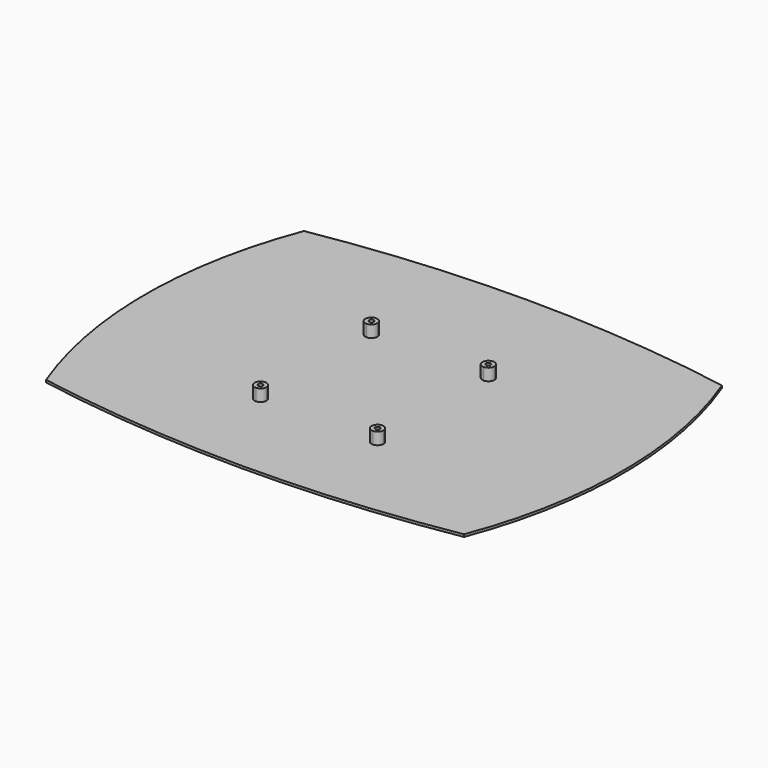
from build123d import *

# Parameters (mm, degrees)
F1_DEPTH        = 1
F3_DEPTH        = 0.5
F5_DEPTH        = 5
F10_D           = 2
F10_DEPTH       = 5
F10_TIP         = 0.600860619
F10_ON_F7_D     = 2
F10_ON_F7_DEPTH = 5
F10_ON_F7_TIP   = 0.600860619
F10_ON_F8_D     = 2
F10_ON_F8_DEPTH = 5
F10_ON_F8_TIP   = 0.600860619
F10_ON_F9_D     = 2
F10_ON_F9_DEPTH = 5
F10_ON_F9_TIP   = 0.600860619


# Not quite as in the source:
# - ends of sketch curves that miss each other by under 0.0002 mm in the source are joined


with BuildPart() as f1:
    # F0 (on Top) → F1 (new body)
    with BuildSketch(Plane.XY):
        with BuildLine():
            ThreePointArc((87.5, -67.5), (100, 0), (87.5, 67.5))
            ThreePointArc((87.5, 67.5), (0, 75), (-87.5, 67.5))
            ThreePointArc((-87.5, 67.5), (-100, 0), (-87.5, -67.5))
            ThreePointArc((-87.5, -67.5), (0, -75), (87.5, -67.5))
        make_face()
    extrude(amount=F1_DEPTH)

    # F2 (on face) → F3 (cut)
    with BuildSketch(Plane(origin=(0, 0, 0), x_dir=(1, 0, 0), z_dir=(0, 0, -1))):
        Polygon((59.9405638027, -1.5313209672), (59.9405638027, -3.714e-05), (59.9405638027, 1.5331036891), (59.6300730728, 6.1295549733), (58.7212563071, 12.0819890983), (57.2441969375, 17.8245820004), (55.2293497966, 23.3313356518), (52.7045699138, 28.5721666207), (49.7021691234, 33.5132774711), (46.2529736583, 38.1275559743), (42.3840957472, 42.3849186981), (38.126361623, 46.2537966092), (33.5117117195, 49.7033634747), (28.5691152675, 52.705764265), (23.3301413005, 55.2305441479), (17.8233876491, 57.2453912888), (12.078937745, 58.7224506584), (6.1268750204, 59.6308960237), (1.5300523358, 59.9395297516), (-0.0008600909, 59.9395297516), (-1.5343723204, 59.9395297516), (-6.1304522042, 59.6308960237), (-12.0828863293, 58.7224506584), (-17.8277076337, 57.2453912888), (-23.3344612852, 55.2305441479), (-28.5734352521, 52.705764265), (-33.5160317041, 49.7033634747), (-38.1304216273, 46.2537966092), (-42.3860387693, 42.3849186981), (-46.2548052603, 38.1275559743), (-49.7044464059, 33.5132774711), (-52.7068100562, 28.5721666207), (-55.2315527989, 23.3313356518), (-57.24651136, 17.8245820004), (-58.7234964495, 12.0819890983), (-59.6322389351, 6.1295549733), (-59.9405384027, 1.5331036891), (-59.9405384027, -3.714e-05), (-59.9405384027, -1.5313209672), (-59.6322389351, -6.127400851), (-58.7234964495, -12.079834976), (-57.24651136, -17.8246562804), (-55.2315527989, -23.3314099319), (-52.7068100562, -28.5722409008), (-49.7044464059, -33.5130917709), (-46.2548052603, -38.1273702741), (-42.3860387693, -42.3850672583), (-38.1284160652, -46.251753907), (-33.5141747021, -49.7034748948), (-28.5734352521, -52.705764265), (-23.3326042832, -55.2285014457), (-17.8254792313, -57.2434600068), (-12.0828863293, -58.7204450962), (-6.1304522042, -59.6291875818), (-1.5343723204, -59.9395297516), (-0.0008600909, -59.9395297516), (1.5300523358, -59.9395297516), (6.1268750204, -59.6291875818), (12.078937745, -58.7204450962), (17.8233876491, -57.2434600068), (23.3301413005, -55.2285014457), (28.5691152675, -52.705764265), (33.5117117195, -49.7034748948), (38.126361623, -46.251753907), (42.3840957472, -42.3850672583), (46.2529736583, -38.1273702741), (49.7021691234, -33.5130917709), (52.7045699138, -28.5722409008), (55.2293497966, -23.3314099319), (57.2441969375, -17.8246562804), (58.7212563071, -12.079834976), (59.6300730728, -6.127400851), align=None)
        Polygon((38.1304470273, -28.6145805458), (15.9292456364, -35.0243199768), (0.9922645644, 2.8311480684), (-20.9062448628, -31.6715753619), (-34.6344668525, -31.6715771942), (-4.051352795, 17.7139046828), (-7.4845780431, 27.4743070541), (-19.3931602971, 27.4743070541), (-19.3931602971, 39.1043390122), (0.9922645644, 39.1043390122), (24.4064596442, -20.4359724552), (34.6987073808, -17.08074129), align=None, mode=Mode.SUBTRACT)
    extrude(amount=-F3_DEPTH, mode=Mode.SUBTRACT)

    # F4 (on face) → F5 (join)
    with BuildSketch(Plane.XY.offset(1)):
        with BuildLine():
            ThreePointArc((-24.5, -31.5), (-26.267766953, -32.232233047), (-27, -34))
            Line((-27, -34), (-24.5, -34))
            Line((-24.5, -34), (-24.5, -31.5))
        make_face()
        with BuildLine():
            Line((-24.5, -31.5), (-24.5, -34))
            Line((-24.5, -34), (-22, -34))
            ThreePointArc((-22, -34), (-22.732233047, -32.232233047), (-24.5, -31.5))
        make_face()
        with BuildLine():
            Line((-22, -34), (-24.5, -34))
            Line((-24.5, -34), (-24.5, -36.5))
            ThreePointArc((-24.5, -36.5), (-22.732233047, -35.767766953), (-22, -34))
        make_face()
        with BuildLine():
            Line((-24.5, -34), (-27, -34))
            ThreePointArc((-27, -34), (-26.267766953, -35.767766953), (-24.5, -36.5))
            Line((-24.5, -36.5), (-24.5, -34))
        make_face()
        with BuildLine():
            Line((-24.5, 24), (-24.5, 26.5))
            ThreePointArc((-24.5, 26.5), (-26.267766953, 25.767766953), (-27, 24))
            Line((-27, 24), (-24.5, 24))
        make_face()
        with BuildLine():
            Line((-24.5, 24), (-27, 24))
            ThreePointArc((-27, 24), (-26.267766953, 22.232233047), (-24.5, 21.5))
            Line((-24.5, 21.5), (-24.5, 24))
        make_face()
        with BuildLine():
            ThreePointArc((-22, 24), (-22.732233047, 25.767766953), (-24.5, 26.5))
            Line((-24.5, 26.5), (-24.5, 24))
            Line((-24.5, 24), (-22, 24))
        make_face()
        with BuildLine():
            Line((-22, 24), (-24.5, 24))
            Line((-24.5, 24), (-24.5, 21.5))
            ThreePointArc((-24.5, 21.5), (-22.732233047, 22.232233047), (-22, 24))
        make_face()
        with BuildLine():
            Line((24.5, -34), (24.5, -31.5))
            ThreePointArc((24.5, -31.5), (22.732233047, -32.232233047), (22, -34))
            Line((22, -34), (24.5, -34))
        make_face()
        with BuildLine():
            ThreePointArc((22, -34), (22.732233047, -35.767766953), (24.5, -36.5))
            Line((24.5, -36.5), (24.5, -34))
            Line((24.5, -34), (22, -34))
        make_face()
        with BuildLine():
            Line((24.5, -34), (27, -34))
            ThreePointArc((27, -34), (26.267766953, -32.232233047), (24.5, -31.5))
            Line((24.5, -31.5), (24.5, -34))
        make_face()
        with BuildLine():
            ThreePointArc((24.5, -36.5), (26.267766953, -35.767766953), (27, -34))
            Line((27, -34), (24.5, -34))
            Line((24.5, -34), (24.5, -36.5))
        make_face()
        with BuildLine():
            Line((24.5, 24), (24.5, 26.5))
            ThreePointArc((24.5, 26.5), (22.732233047, 25.767766953), (22, 24))
            Line((22, 24), (24.5, 24))
        make_face()
        with BuildLine():
            ThreePointArc((27, 24), (26.267766953, 25.767766953), (24.5, 26.5))
            Line((24.5, 26.5), (24.5, 24))
            Line((24.5, 24), (27, 24))
        make_face()
        with BuildLine():
            Line((27, 24), (24.5, 24))
            Line((24.5, 24), (24.5, 21.5))
            ThreePointArc((24.5, 21.5), (26.267766953, 22.232233047), (27, 24))
        make_face()
        with BuildLine():
            Line((24.5, 21.5), (24.5, 24))
            Line((24.5, 24), (22, 24))
            ThreePointArc((22, 24), (22.732233047, 22.232233047), (24.5, 21.5))
        make_face()
    extrude(amount=F5_DEPTH)

    # F10
    with Locations(Plane.XY.offset(6)):
        with Locations((-24.5, 24)):
            Hole(F10_D / 2, depth=F10_DEPTH)
            with Locations((0, 0, -(F10_DEPTH + F10_TIP / 2))):  # 118° drill point
                Cone(0, F10_D / 2, F10_TIP, mode=Mode.SUBTRACT)

    # F10 on F7
    with Locations(Plane.XY.offset(6)):
        with Locations((24.5, 24)):
            Hole(F10_ON_F7_D / 2, depth=F10_ON_F7_DEPTH)
            with Locations((0, 0, -(F10_ON_F7_DEPTH + F10_ON_F7_TIP / 2))):  # 118° drill point
                Cone(0, F10_ON_F7_D / 2, F10_ON_F7_TIP, mode=Mode.SUBTRACT)

    # F10 on F8
    with Locations(Plane.XY.offset(6)):
        with Locations((-24.5, -34)):
            Hole(F10_ON_F8_D / 2, depth=F10_ON_F8_DEPTH)
            with Locations((0, 0, -(F10_ON_F8_DEPTH + F10_ON_F8_TIP / 2))):  # 118° drill point
                Cone(0, F10_ON_F8_D / 2, F10_ON_F8_TIP, mode=Mode.SUBTRACT)

    # F10 on F9
    with Locations(Plane.XY.offset(6)):
        with Locations((24.5, -34)):
            Hole(F10_ON_F9_D / 2, depth=F10_ON_F9_DEPTH)
            with Locations((0, 0, -(F10_ON_F9_DEPTH + F10_ON_F9_TIP / 2))):  # 118° drill point
                Cone(0, F10_ON_F9_D / 2, F10_ON_F9_TIP, mode=Mode.SUBTRACT)


solid = f1.part
